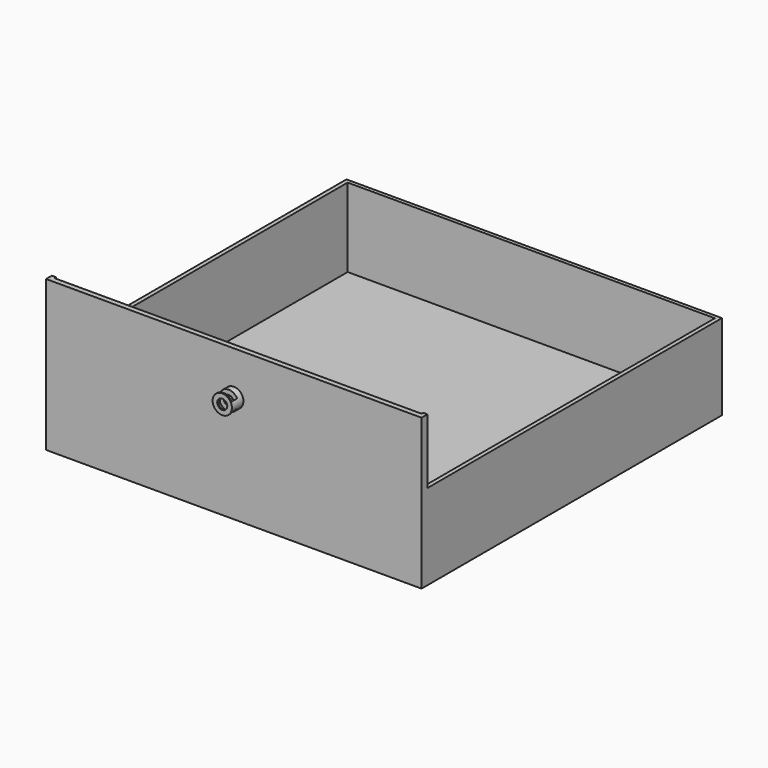
from build123d import *

# Parameters (mm, degrees)
F0_W      = 125.476
F0_H      = 50.292
F1_DEPTH  = 125.476
F2_W      = 122.7189972997
F2_H      = 122.4945134018
F3_DEPTH  = 48.006
F5_R      = 3.2177672419
F5_R_2    = 1.6781805888
F6_DEPTH  = 4.826
F7_W      = 80.5568695068
F7_H      = 21.6923308617
F8_DEPTH  = 125.477
F9_W      = 42.4876958132
F9_H      = 25.0391000882
F10_DEPTH = 125.477
F11_W     = 5.6567939464
F11_H     = 2.2512227297
F12_DEPTH = 48.007


# Not quite as in the source:
# - a feature names something its author has since deleted; it is built from what else it names


with BuildPart() as f1:
    # F0 (on Front) → F1 (new body)
    with BuildSketch(Plane.XZ):
        Rectangle(F0_W, F0_H)
    extrude(amount=F1_DEPTH)

    # F2 (on face) → F3 (cut)
    with BuildSketch(Plane.XY.offset(25.146)):
        with Locations((7.4506e-06, -62.4770697905)):
            Rectangle(F2_W, F2_H)
    extrude(amount=-F3_DEPTH, mode=Mode.SUBTRACT)

    # F5 (on face) → F6 (join)
    with BuildSketch(Plane.XZ.offset(125.476)):
        with Locations((0, 10.6488130987)):
            Circle(F5_R)
        with Locations((0, 10.6488130987)):
            Circle(F5_R_2, mode=Mode.SUBTRACT)
    extrude(amount=F6_DEPTH)

    # F7 (on face) → F8 (cut, through all)
    with BuildSketch(Plane.YZ.offset(62.738)):
        with Locations((-40.2784347534, 14.2998345691)):
            Rectangle(F7_W, F7_H)
    extrude(amount=-F8_DEPTH, mode=Mode.SUBTRACT)

    # F9 (on face) → F10 (cut, through all)
    with BuildSketch(Plane.YZ.offset(62.738)):
        with Locations((-101.8007174134, 15.9732191823)):
            Rectangle(F9_W, F9_H)
    extrude(amount=-F10_DEPTH, mode=Mode.SUBTRACT)

    # F11 (on face) → F12 (cut, through all)
    with BuildSketch(Plane.XY.offset(-22.86)):
        with Locations((-0.0043596374, -128.7486031651)):
            Rectangle(F11_W, F11_H)
    extrude(amount=F12_DEPTH, mode=Mode.SUBTRACT)


solid = f1.part
